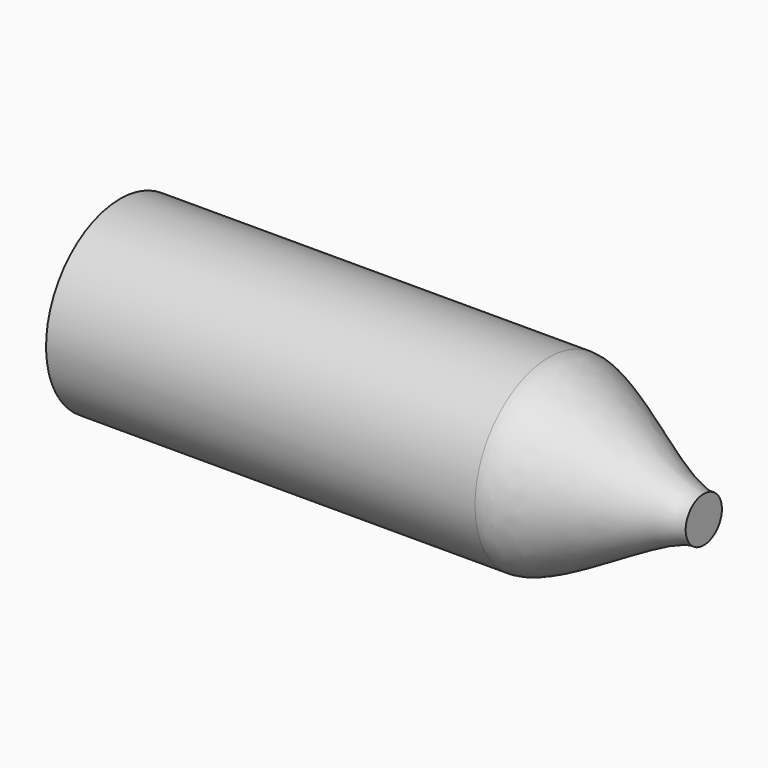
from build123d import *


# Not quite as in the source:
# - ends of sketch curves that miss each other by under 0.0002 mm in the source are joined
# - the dataset's text gives a spline's control points without its knots; the knots are read off the source's solid


with BuildPart() as f1:
    # F0 (on Front) → F1 (revolve)
    with BuildSketch(Plane.XZ):
        with BuildLine():
            Line((37.4922007322, 0), (39.4921973348, 0))
            Line((39.4921973348, 0), (39.4921973348, 10.6321773492))
            add(Edge.make_bspline(
                [(39.4921973348, 10.6321773492), (25.8319638669, 9.223905392), (-17.5490600107, 43.4075947851), (-33.0458087847, 43.4075947851)],
                knots=[0, 0, 0, 0, 79.598934163, 79.598934163, 79.598934163, 79.598934163], degree=3))
            Line((-33.0458087847, 43.4075947851), (-234.167508781, 43.4075947851))
            Line((-234.167508781, 43.4075947851), (-234.167508781, 0))
            Line((-234.167508781, 0), (-232.1675121784, 0))
            Line((-232.1675121784, 0), (-232.1675121784, 41.4075981826))
            Line((-232.1675121784, 41.4075981826), (-33.0458087847, 41.4075981826))
            add(Edge.make_bspline(
                [(37.4922013196, 8.6412238335), (37.0945770822, 8.6758484487), (35.5138249558, 8.8768940457), (32.5543086746, 9.6271891204), (28.3485189273, 11.2022557551), (22.229588287, 13.9850146115), (13.76876914, 18.4938124906), (2.9175771692, 24.7537479723), (-7.9699760264, 31.0509027544), (-16.502875169, 35.6449766342), (-22.6377369359, 38.5118930501), (-26.788697304, 40.1529468803), (-30.3678361719, 41.1839581397), (-32.2610835082, 41.4075981826), (-33.0458087847, 41.4075981826)],
                knots=[0.0410074938, 0.0410074938, 0.0410074938, 0.0410074938, 0.0625, 0.125, 0.1875, 0.25, 0.375, 0.5, 0.625, 0.75, 0.8125, 0.875, 0.9375, 1, 1, 1, 1], degree=3))
            Line((37.4922013196, 8.6412238335), (37.4922007322, 0))
        make_face()
    revolve(axis=Axis((-25.0741094351, 0, 0), (1, 0, 0)))


solid = f1.part
